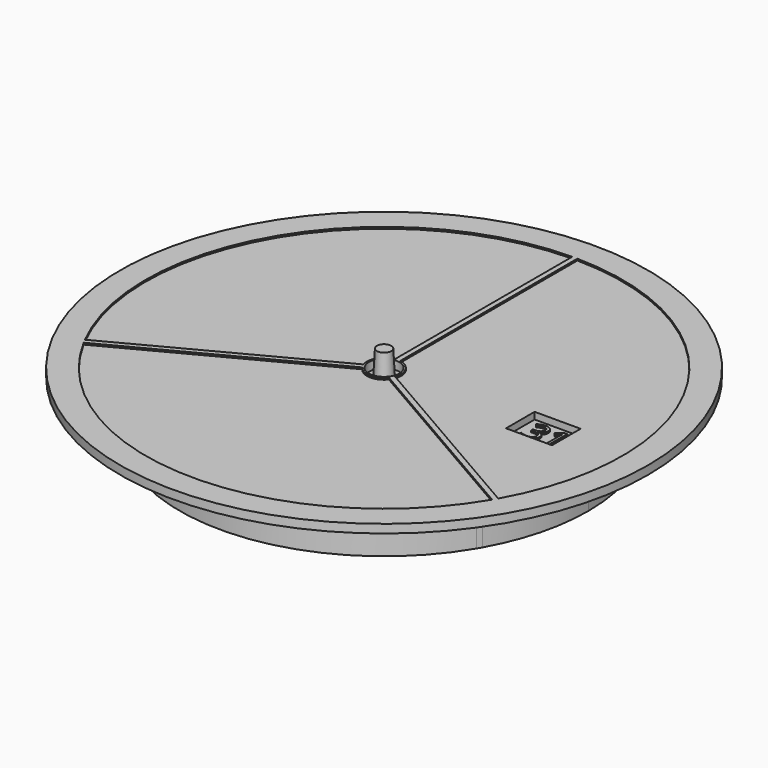
from build123d import *

# Parameters (mm, degrees)
F0_W         = 2.7
F0_H         = 2.1
F0_R         = 0.9
F0_R_2       = 0.5
F0_TEXT_SIZE = 1.9855353457
F1_DEPTH     = 3
F0_R_3       = 15.5
F2_DEPTH     = 0.5
F3_DEPTH     = 0.4
F4_DEPTH     = 1.5
F4_TAPER     = 3
F5_DEPTH     = 0.1


# Not quite as in the source:
# - Text() gives the source's letters only with a copy of the font that has no kerning and outlines rounded to 1/6400 em; it was checked with that copy


with BuildPart() as f1:
    # F0 (on Top) → F1 (new body)
    with BuildSketch(Plane.XY):
        with BuildLine():
            ThreePointArc((-10.5444954952, -5.7283169214), (-0.2306951037, -11.9977822855), (10.3164929149, -6.1294350423))
            Line((10.3164929149, -6.1294350423), (0.7812271895, -0.6242468089))
            ThreePointArc((0.7812271895, -0.6242468089), (-0.0192242884, -0.9998151963), (-0.804646714, -0.5937538763))
            Line((-0.804646714, -0.5937538763), (-10.5444954952, -5.7283169214))
        make_face()
        with BuildLine():
            Line((0.9312271895, -0.3644391878), (10.4664929149, -5.8696274211))
            ThreePointArc((10.4664929149, -5.8696274211), (11.6102953231, -3.0333220256), (12, 0))
            ThreePointArc((12, 0), (8.5381471226, 8.4320841856), (0.1499927145, 11.9990625544))
            Line((0.1499927145, 11.9990625544), (0.15, 0.9886859967))
            ThreePointArc((0.15, 0.9886859967), (0.8660254038, 0.5), (0.9312271895, -0.3644391878))
        make_face()
        with Locations((9.35, 0)):
            Rectangle(F0_W, F0_H, mode=Mode.SUBTRACT)
        with BuildLine():
            Line((-0.15, 0.9886859967), (-0.1499927145, 11.9990625544))
            ThreePointArc((-0.1499927145, 11.9990625544), (-10.2750385782, 6.1986758437), (-10.684390441, -5.462948005))
            Line((-10.684390441, -5.462948005), (-0.9445484548, -0.3283720704))
            ThreePointArc((-0.9445484548, -0.3283720704), (-0.8562532149, 0.5165563203), (-0.15, 0.9886859967))
        make_face()
        with BuildLine():
            ThreePointArc((10.3164929149, -6.1294350423), (10.3923048454, -6), (10.4664929149, -5.8696274211))
            Line((10.4664929149, -5.8696274211), (0.9312271895, -0.3644391878))
            ThreePointArc((0.9312271895, -0.3644391878), (0.8660254038, 0.5), (0.15, 0.9886859967))
            Line((0.15, 0.9886859967), (0.1499927145, 11.9990625544))
            ThreePointArc((0.1499927145, 11.9990625544), (0, 12), (-0.1499927145, 11.9990625544))
            Line((-0.1499927145, 11.9990625544), (-0.15, 0.9886859967))
            ThreePointArc((-0.15, 0.9886859967), (-0.8562532149, 0.5165563203), (-0.9445484548, -0.3283720704))
            Line((-0.9445484548, -0.3283720704), (-10.684390441, -5.462948005))
            ThreePointArc((-10.684390441, -5.462948005), (-10.6152722381, -5.5960696307), (-10.5444954952, -5.7283169214))
            Line((-10.5444954952, -5.7283169214), (-0.804646714, -0.5937538763))
            ThreePointArc((-0.804646714, -0.5937538763), (-0.0192242884, -0.9998151963), (0.7812271895, -0.6242468089))
            Line((0.7812271895, -0.6242468089), (10.3164929149, -6.1294350423))
        make_face()
        Circle(F0_R, mode=Mode.SUBTRACT)
        with Locations((9.35, 0)):
            Rectangle(F0_W, F0_H)
        with BuildLine():
            add(Edge.make_bspline(
                [(9.2201225567, 0.6365668483), (9.334601079, 0.5420987994), (9.334601079, 0.3773614137)],
                knots=[0, 0, 0, 1, 1, 1], degree=2))
            add(Edge.make_bspline(
                [(9.334601079, 0.3773614137), (9.334601079, 0.2414763385), (9.2584371841, 0.1552296469)],
                knots=[0, 0, 0, 1, 1, 1], degree=2))
            add(Edge.make_bspline(
                [(9.2584371841, 0.1552296469), (9.1822732892, 0.0689829553), (9.0426653352, 0.0398204049)],
                knots=[0, 0, 0, 1, 1, 1], degree=2))
            Line((9.0426653352, 0.0398204049), (9.0426653352, 0.0320644075))
            add(Edge.make_bspline(
                [(9.0426653352, 0.0320644075), (9.213297279, 0.0109680944), (9.2956659718, -0.0763644368)],
                knots=[0, 0, 0, 1, 1, 1], degree=2))
            add(Edge.make_bspline(
                [(9.2956659718, -0.0763644368), (9.3780346647, -0.163696968), (9.3780346647, -0.3051663614)],
                knots=[0, 0, 0, 1, 1, 1], degree=2))
            add(Edge.make_bspline(
                [(9.3780346647, -0.3051663614), (9.3780346647, -0.5077530146), (9.237495991, -0.6169574586)],
                knots=[0, 0, 0, 1, 1, 1], degree=2))
            add(Edge.make_bspline(
                [(9.237495991, -0.6169574586), (9.0969573173, -0.7261619027), (8.8382172426, -0.7261619027)],
                knots=[0, 0, 0, 1, 1, 1], degree=2))
            add(Edge.make_bspline(
                [(8.8382172426, -0.7261619027), (8.7256001597, -0.7261619027), (8.6320628305, -0.7090987083)],
                knots=[0, 0, 0, 1, 1, 1], degree=2))
            add(Edge.make_bspline(
                [(8.6320628305, -0.7090987083), (8.5385255013, -0.6920355139), (8.4504173703, -0.6495326479)],
                knots=[0, 0, 0, 1, 1, 1], degree=2))
            Line((8.4504173703, -0.6495326479), (8.4504173703, -0.4962741384))
            add(Edge.make_bspline(
                [(8.4504173703, -0.4962741384), (8.54255862, -0.5418794034), (8.6467992256, -0.5656127556)],
                knots=[0, 0, 0, 1, 1, 1], degree=2))
            add(Edge.make_bspline(
                [(8.6467992256, -0.5656127556), (8.7510398313, -0.5893461077), (8.8441118006, -0.5893461077)],
                knots=[0, 0, 0, 1, 1, 1], degree=2))
            add(Edge.make_bspline(
                [(8.8441118006, -0.5893461077), (9.2114358396, -0.5893461077), (9.2114358396, -0.3014434826)],
                knots=[0, 0, 0, 1, 1, 1], degree=2))
            add(Edge.make_bspline(
                [(9.2114358396, -0.3014434826), (9.2114358396, -0.0433238877), (8.8062625331, -0.0433238877)],
                knots=[0, 0, 0, 1, 1, 1], degree=2))
            Line((8.8062625331, -0.0433238877), (8.6666545791, -0.0433238877))
            Line((8.6666545791, -0.0433238877), (8.6666545791, 0.0950431067))
            Line((8.6666545791, 0.0950431067), (8.8081239725, 0.0950431067))
            add(Edge.make_bspline(
                [(8.8081239725, 0.0950431067), (8.9737920779, 0.0950431067), (9.0707420459, 0.1682597226)],
                knots=[0, 0, 0, 1, 1, 1], degree=2))
            add(Edge.make_bspline(
                [(9.0707420459, 0.1682597226), (9.167692014, 0.2414763385), (9.167692014, 0.3714668557)],
                knots=[0, 0, 0, 1, 1, 1], degree=2))
            add(Edge.make_bspline(
                [(9.167692014, 0.3714668557), (9.167692014, 0.4750869815), (9.0964919575, 0.534342802)],
                knots=[0, 0, 0, 1, 1, 1], degree=2))
            add(Edge.make_bspline(
                [(9.0964919575, 0.534342802), (9.0252919009, 0.5935986225), (8.9030573812, 0.5935986225)],
                knots=[0, 0, 0, 1, 1, 1], degree=2))
            add(Edge.make_bspline(
                [(8.9030573812, 0.5935986225), (8.8099854119, 0.5935986225), (8.727616719, 0.5683140708)],
                knots=[0, 0, 0, 1, 1, 1], degree=2))
            add(Edge.make_bspline(
                [(8.727616719, 0.5683140708), (8.6452480261, 0.5430295191), (8.539456221, 0.4750869815)],
                knots=[0, 0, 0, 1, 1, 1], degree=2))
            Line((8.539456221, 0.4750869815), (8.4581733678, 0.5836709457))
            add(Edge.make_bspline(
                [(8.4581733678, 0.5836709457), (8.5453507791, 0.652544203), (8.6592088215, 0.6917895501)],
                knots=[0, 0, 0, 1, 1, 1], degree=2))
            add(Edge.make_bspline(
                [(8.6592088215, 0.6917895501), (8.773066864, 0.7310348972), (8.8993345024, 0.7310348972)],
                knots=[0, 0, 0, 1, 1, 1], degree=2))
            add(Edge.make_bspline(
                [(8.8993345024, 0.7310348972), (9.1056440344, 0.7310348972), (9.2201225567, 0.6365668483)],
                knots=[0, 0, 0, 1, 1, 1], degree=2))
        make_face(mode=Mode.SUBTRACT)
        with BuildLine():
            Line((10.187450558, 0.7108693038), (10.187450558, -0.7066167891))
            Line((10.187450558, -0.7066167891), (10.0304691697, -0.7066167891))
            Line((10.0304691697, -0.7066167891), (10.0304691697, 0.303524318))
            add(Edge.make_bspline(
                [(10.0304691697, 0.303524318), (10.0304691697, 0.4297919564), (10.0382251671, 0.5420987994)],
                knots=[0, 0, 0, 1, 1, 1], degree=2))
            add(Edge.make_bspline(
                [(10.0382251671, 0.5420987994), (10.0180595738, 0.5216229662), (9.9927750221, 0.4994408135)],
                knots=[0, 0, 0, 1, 1, 1], degree=2))
            add(Edge.make_bspline(
                [(9.9927750221, 0.4994408135), (9.9674904704, 0.4772586608), (9.7621116581, 0.3103495958)],
                knots=[0, 0, 0, 1, 1, 1], degree=2))
            Line((9.7621116581, 0.3103495958), (9.6767956862, 0.4207949994))
            Line((9.6767956862, 0.4207949994), (10.0518757226, 0.7108693038))
            Line((10.0518757226, 0.7108693038), (10.187450558, 0.7108693038))
        make_face(mode=Mode.SUBTRACT)
        Circle(F0_R)
        Circle(F0_R_2, mode=Mode.SUBTRACT)
        with Locations((8.3592068404, -0.7066167891)):
            Text('31', F0_TEXT_SIZE, font='Open Sans', text_align=(TextAlign.LEFT, TextAlign.BOTTOM))
    extrude(amount=-F1_DEPTH)

    # F0 (on Top) → F5 (join)
    with BuildSketch(Plane.XY):
        with Locations((8.3592068404, -0.7066167891)):
            Text('31', F0_TEXT_SIZE, font='Open Sans', text_align=(TextAlign.LEFT, TextAlign.BOTTOM))
    extrude(amount=F5_DEPTH)


with BuildPart() as f2:
    # F0 (on Top) → F2 (new body)
    with BuildSketch(Plane.XY):
        Circle(F0_R_3)
        with BuildLine():
            ThreePointArc((0.149991391, 13.9991964977), (12.1243535006, 7.000003728), (12.1986597197, -6.8696943922))
            Line((12.1986597197, -6.8696943922), (10.4664929149, -5.8696274211))
            ThreePointArc((10.4664929149, -5.8696274211), (10.3923048454, -6), (10.3164929149, -6.1294350423))
            Line((10.3164929149, -6.1294350423), (12.0486597197, -7.1295020133))
            ThreePointArc((12.0486597197, -7.1295020133), (-0.2691443422, -13.9974126653), (-12.3138266391, -6.6610564854))
            Line((-12.3138266391, -6.6610564854), (-10.5444954952, -5.7283169214))
            ThreePointArc((-10.5444954952, -5.7283169214), (-10.6152722381, -5.5960696307), (-10.684390441, -5.462948005))
            Line((-10.684390441, -5.462948005), (-12.4537203505, -6.3956899105))
            ThreePointArc((-12.4537203505, -6.3956899105), (-11.987545008, 7.2317884843), (-0.149991391, 13.9991964977))
            Line((-0.149991391, 13.9991964977), (-0.1499927145, 11.9990625544))
            ThreePointArc((-0.1499927145, 11.9990625544), (0, 12), (0.1499927145, 11.9990625544))
            Line((0.1499927145, 11.9990625544), (0.149991391, 13.9991964977))
        make_face(mode=Mode.SUBTRACT)
        with BuildLine():
            ThreePointArc((10.3164929149, -6.1294350423), (10.3923048454, -6), (10.4664929149, -5.8696274211))
            Line((10.4664929149, -5.8696274211), (0.9312271895, -0.3644391878))
            ThreePointArc((0.9312271895, -0.3644391878), (0.8660254038, 0.5), (0.15, 0.9886859967))
            Line((0.15, 0.9886859967), (0.1499927145, 11.9990625544))
            ThreePointArc((0.1499927145, 11.9990625544), (0, 12), (-0.1499927145, 11.9990625544))
            Line((-0.1499927145, 11.9990625544), (-0.15, 0.9886859967))
            ThreePointArc((-0.15, 0.9886859967), (-0.8562532149, 0.5165563203), (-0.9445484548, -0.3283720704))
            Line((-0.9445484548, -0.3283720704), (-10.684390441, -5.462948005))
            ThreePointArc((-10.684390441, -5.462948005), (-10.6152722381, -5.5960696307), (-10.5444954952, -5.7283169214))
            Line((-10.5444954952, -5.7283169214), (-0.804646714, -0.5937538763))
            ThreePointArc((-0.804646714, -0.5937538763), (-0.0192242884, -0.9998151963), (0.7812271895, -0.6242468089))
            Line((0.7812271895, -0.6242468089), (10.3164929149, -6.1294350423))
        make_face()
        Circle(F0_R, mode=Mode.SUBTRACT)
    extrude(amount=F2_DEPTH)


with BuildPart() as f3:
    # F0 (on Top) → F3 (new body)
    with BuildSketch(Plane.XY):
        with BuildLine():
            Line((10.4664929149, -5.8696274211), (12.1986597197, -6.8696943922))
            ThreePointArc((12.1986597197, -6.8696943922), (12.1243535006, 7.000003728), (0.149991391, 13.9991964977))
            Line((0.149991391, 13.9991964977), (0.1499927145, 11.9990625544))
            ThreePointArc((0.1499927145, 11.9990625544), (8.5381471226, 8.4320841856), (12, 0))
            ThreePointArc((12, 0), (11.6102953231, -3.0333220256), (10.4664929149, -5.8696274211))
        make_face()
        with BuildLine():
            Line((0.9312271895, -0.3644391878), (10.4664929149, -5.8696274211))
            ThreePointArc((10.4664929149, -5.8696274211), (11.6102953231, -3.0333220256), (12, 0))
            ThreePointArc((12, 0), (8.5381471226, 8.4320841856), (0.1499927145, 11.9990625544))
            Line((0.1499927145, 11.9990625544), (0.15, 0.9886859967))
            ThreePointArc((0.15, 0.9886859967), (0.8660254038, 0.5), (0.9312271895, -0.3644391878))
        make_face()
        with Locations((9.35, 0)):
            Rectangle(F0_W, F0_H, mode=Mode.SUBTRACT)
    extrude(amount=F3_DEPTH)


with BuildPart() as f3b:
    # F0 (on Top) → F3, piece 2 (new body)
    with BuildSketch(Plane.XY):
        with BuildLine():
            ThreePointArc((-10.684390441, -5.462948005), (-10.2750385782, 6.1986758437), (-0.1499927145, 11.9990625544))
            Line((-0.1499927145, 11.9990625544), (-0.149991391, 13.9991964977))
            ThreePointArc((-0.149991391, 13.9991964977), (-11.987545008, 7.2317884843), (-12.4537203505, -6.3956899105))
            Line((-12.4537203505, -6.3956899105), (-10.684390441, -5.462948005))
        make_face()
        with BuildLine():
            Line((-0.15, 0.9886859967), (-0.1499927145, 11.9990625544))
            ThreePointArc((-0.1499927145, 11.9990625544), (-10.2750385782, 6.1986758437), (-10.684390441, -5.462948005))
            Line((-10.684390441, -5.462948005), (-0.9445484548, -0.3283720704))
            ThreePointArc((-0.9445484548, -0.3283720704), (-0.8562532149, 0.5165563203), (-0.15, 0.9886859967))
        make_face()
    extrude(amount=F3_DEPTH)


with BuildPart() as f3c:
    # F0 (on Top) → F3, piece 3 (new body)
    with BuildSketch(Plane.XY):
        with BuildLine():
            ThreePointArc((-10.5444954952, -5.7283169214), (-0.2306951037, -11.9977822855), (10.3164929149, -6.1294350423))
            Line((10.3164929149, -6.1294350423), (0.7812271895, -0.6242468089))
            ThreePointArc((0.7812271895, -0.6242468089), (-0.0192242884, -0.9998151963), (-0.804646714, -0.5937538763))
            Line((-0.804646714, -0.5937538763), (-10.5444954952, -5.7283169214))
        make_face()
        with BuildLine():
            Line((12.0486597197, -7.1295020133), (10.3164929149, -6.1294350423))
            ThreePointArc((10.3164929149, -6.1294350423), (-0.2306951037, -11.9977822855), (-10.5444954952, -5.7283169214))
            Line((-10.5444954952, -5.7283169214), (-12.3138266391, -6.6610564854))
            ThreePointArc((-12.3138266391, -6.6610564854), (-0.2691443422, -13.9974126653), (12.0486597197, -7.1295020133))
        make_face()
    extrude(amount=F3_DEPTH)


with BuildPart() as f4:
    # F0 (on Top) → F4 (new body)
    with BuildSketch(Plane.XY):
        Circle(F0_R_2)
    extrude(amount=F4_DEPTH, taper=F4_TAPER)


solid = Compound([f1.part, f2.part, f3.part, f3b.part, f3c.part, f4.part])
